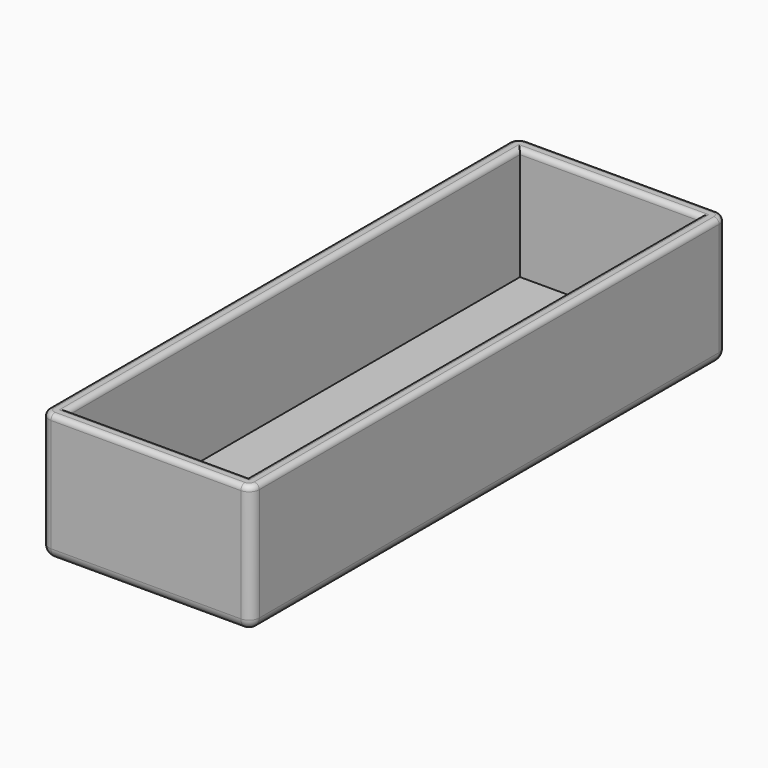
from build123d import *

# Parameters (mm, degrees)
F0_W         = 35
F0_H         = 110
F1_DEPTH     = 3
F2_W         = 41
F2_H         = 116
F2_W_2       = 35
F2_H_2       = 110
F3_DEPTH     = 25
F4_R         = 1
F5_T1_DEPTH  = 30
F5_T4_ANGLE  = 90
F5_T6_ANGLE  = 90
F5_T8_ANGLE  = 90
F5_T10_ANGLE = 90
F7_W         = 100
F7_H         = 1
F8_DEPTH     = 1
F9_R         = 2


# Not quite as in the source:
# - a fillet or chamfer that OpenCascade refuses, or shapes differently, is made with other operations: its cross-section is extruded or revolved along the edge and cut away or added


with BuildPart() as f1:
    # F0 (on Top) → F1 (new body)
    with BuildSketch(Plane.XY):
        Rectangle(F0_W, F0_H)
    extrude(amount=F1_DEPTH)

    # F2 (on Top) → F3 (join)
    with BuildSketch(Plane.XY):
        Rectangle(F2_W, F2_H)
        Rectangle(F2_W_2, F2_H_2, mode=Mode.SUBTRACT)
    extrude(amount=F3_DEPTH)

    # F4
    f4_edges = [f1.edges().sort_by_distance(p)[0] for p in [
        (20.5, 0, 25),
        (0, 58, 25),
        (-20.5, 0, 25),
        (0, -58, 25),
        (-17.5, 0, 25),
        (0, 55, 25),
        (17.5, 0, 25),
        (0, -55, 25),
    ]]
    fillet(f4_edges, radius=F4_R)

    # F5: fillet of radius 2 on 4 edges, made by hand

    # F5_s2 → F5_t1 (cut)
    with BuildSketch(Plane.XY.offset(-5)):
        with BuildLine():
            ThreePointArc((20.5, -56), (19.9142135624, -57.4142135624), (18.5, -58))
            Line((18.5, -58), (20.5, -58))
            Line((20.5, -58), (20.5, -56))
        make_face()
        with BuildLine():
            ThreePointArc((-18.5, -58), (-19.9142135624, -57.4142135624), (-20.5, -56))
            Line((-20.5, -56), (-20.5, -58))
            Line((-20.5, -58), (-18.5, -58))
        make_face()
        with BuildLine():
            ThreePointArc((-18.5, 58), (-19.9142135624, 57.4142135624), (-20.5, 56))
            Line((-20.5, 56), (-20.5, 58))
            Line((-20.5, 58), (-18.5, 58))
        make_face()
        with BuildLine():
            ThreePointArc((20.5, 56), (19.9142135624, 57.4142135624), (18.5, 58))
            Line((18.5, 58), (20.5, 58))
            Line((20.5, 58), (20.5, 56))
        make_face()
    extrude(amount=F5_T1_DEPTH, mode=Mode.SUBTRACT)

    # F5_s3 → F5_t4 (revolve, cut)
    with BuildSketch(Plane.XZ.offset(-56)):
        with BuildLine():
            ThreePointArc((19.5, 25), (20.2071067812, 24.7071067812), (20.5, 24))
            Line((20.5, 24), (20.5, 25))
            Line((20.5, 25), (19.5, 25))
        make_face()
    revolve(axis=Axis((18.5, 56, 25), (0, 0, 1)), revolution_arc=F5_T4_ANGLE, mode=Mode.SUBTRACT)

    # F5_s5 → F5_t6 (revolve, cut)
    with BuildSketch(Plane.YZ.offset(-18.5)):
        with BuildLine():
            ThreePointArc((57, 25), (57.7071067812, 24.7071067812), (58, 24))
            Line((58, 24), (58, 25))
            Line((58, 25), (57, 25))
        make_face()
    revolve(axis=Axis((-18.5, 56, 25), (0, 0, 1)), revolution_arc=F5_T6_ANGLE, mode=Mode.SUBTRACT)

    # F5_s7 → F5_t8 (revolve, cut)
    with BuildSketch(Plane.XZ.offset(56)):
        with BuildLine():
            ThreePointArc((-19.5, 25), (-20.2071067812, 24.7071067812), (-20.5, 24))
            Line((-20.5, 24), (-20.5, 25))
            Line((-20.5, 25), (-19.5, 25))
        make_face()
    revolve(axis=Axis((-18.5, -56, 25), (0, 0, 1)), revolution_arc=F5_T8_ANGLE, mode=Mode.SUBTRACT)

    # F5_s9 → F5_t10 (revolve, cut)
    with BuildSketch(Plane.YZ.offset(18.5)):
        with BuildLine():
            ThreePointArc((-57, 25), (-57.7071067812, 24.7071067812), (-58, 24))
            Line((-58, 24), (-58, 25))
            Line((-58, 25), (-57, 25))
        make_face()
    revolve(axis=Axis((18.5, -56, 25), (0, 0, 1)), revolution_arc=F5_T10_ANGLE, mode=Mode.SUBTRACT)

    # F7 (on face) → F8 (cut)
    with BuildSketch(Plane(origin=(-20.5, 0, 0), x_dir=(0, -1, 0), z_dir=(-1, 0, 0))):
        with Locations((-0.0301606953, 18.6210061312)):
            Rectangle(F7_W, F7_H)
    extrude(amount=-F8_DEPTH, mode=Mode.SUBTRACT)

    # F9
    f9_edges = [f1.edges().sort_by_distance(p)[0] for p in [
        (19.914214, -57.414214, 0),
        (0, -58, 0),
        (-19.914214, -57.414214, 0),
        (-20.5, 0, 0),
        (-19.914214, 57.414214, 0),
        (0, 58, 0),
        (19.914214, 57.414214, 0),
        (20.5, 0, 0),
    ]]
    fillet(f9_edges, radius=F9_R)


solid = f1.part
